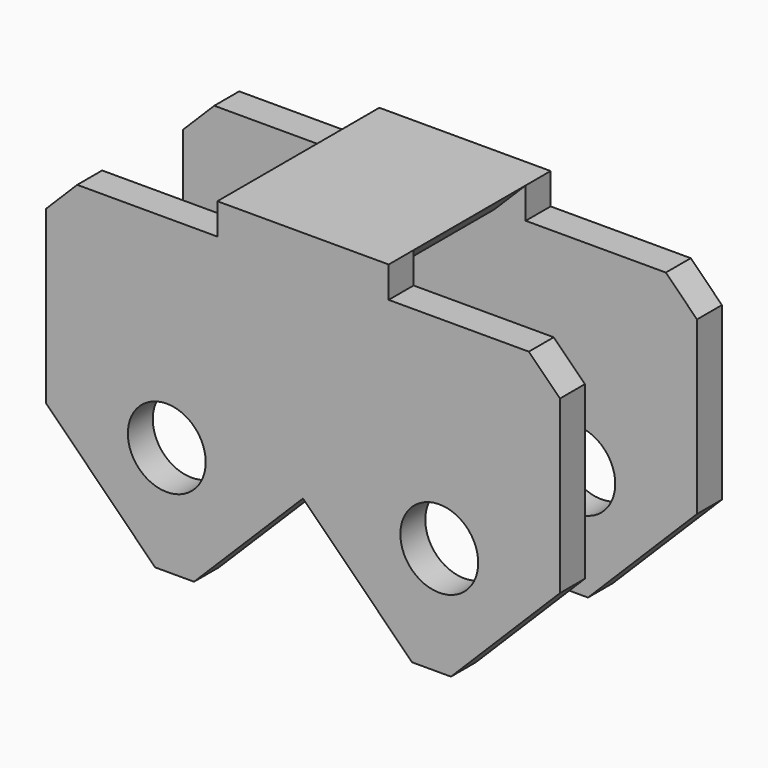
from build123d import *

# Parameters (mm, degrees)
F0_W      = 33
F0_H      = 22
F2_DEPTH  = 13
F3_SIZE   = 7
F4_R      = 2.5
F5_DEPTH  = 25
F6_T      = -2
F7_W      = 11
F7_H      = 13
F8_DEPTH  = 2
F9_SIZE   = 1.99999
F11_DEPTH = 25
F12_SIZE  = 2


# Not quite as in the source:
# - a fillet or chamfer is up to 0.001 mm smaller than in the source, because OpenCascade refuses the exact size


with BuildPart() as f2:
    # F0 (on Front) → F2 (new body)
    with BuildSketch(Plane.XZ):
        Rectangle(F0_W, F0_H)
    extrude(amount=F2_DEPTH)

    # F3
    f3_edges = [f2.edges().sort_by_distance(p)[0] for p in [
        (-16.5, -6.5, -11),
        (16.5, -6.5, -11),
    ]]
    chamfer(f3_edges, length=F3_SIZE)

    # F4 (on face) → F5 (cut)
    with BuildSketch(Plane.XZ.offset(13)):
        with Locations((-8.75, -4)):
            Circle(F4_R)
        with Locations((8.75, -4)):
            Circle(F4_R)
    extrude(amount=-F5_DEPTH, mode=Mode.SUBTRACT)

    # F6
    f6_openings = [f2.faces().sort_by_distance(p)[0] for p in [
        (0, -6.5, -11),
        (13, -6.5, -7.5),
        (16.5, -6.5, 3.5),
        (-16.5, -6.5, 3.5),
        (-13, -6.5, -7.5),
        (-11.25, -6.5, -4),
        (6.25, -6.5, -4),
    ]]
    offset(amount=F6_T, openings=f6_openings)

    # F7 (on face) → F8 (cut)
    with BuildSketch(Plane.XY.offset(11)):
        with Locations((11, -6.5)):
            Rectangle(F7_W, F7_H)
        with Locations((-11, -6.5)):
            Rectangle(F7_W, F7_H)
    extrude(amount=-F8_DEPTH, mode=Mode.SUBTRACT)

    # F9 (size 2 in the source; OpenCascade refuses exactly that, so slightly less here)
    f9_edges = [f2.edges().sort_by_distance(p)[0] for p in [
        (5.5, -6.5, 9),
        (-5.5, -6.5, 9),
    ]]
    chamfer(f9_edges, length=F9_SIZE)

    # F10 (on face) → F11 (cut)
    with BuildSketch(Plane(origin=(0, 0, 0), x_dir=(-1, 0, 0), z_dir=(0, 1, 0))):
        Polygon((7, -11), (0, -4.0134343201), (-7, -11), align=None)
    extrude(amount=-F11_DEPTH, mode=Mode.SUBTRACT)

    # F12
    f12_edges = [f2.edges().sort_by_distance(p)[0] for p in [
        (16.5, -12, 9),
        (16.5, -1, 9),
        (-16.5, -12, 9),
        (-16.5, -1, 9),
    ]]
    chamfer(f12_edges, length=F12_SIZE)


solid = f2.part
